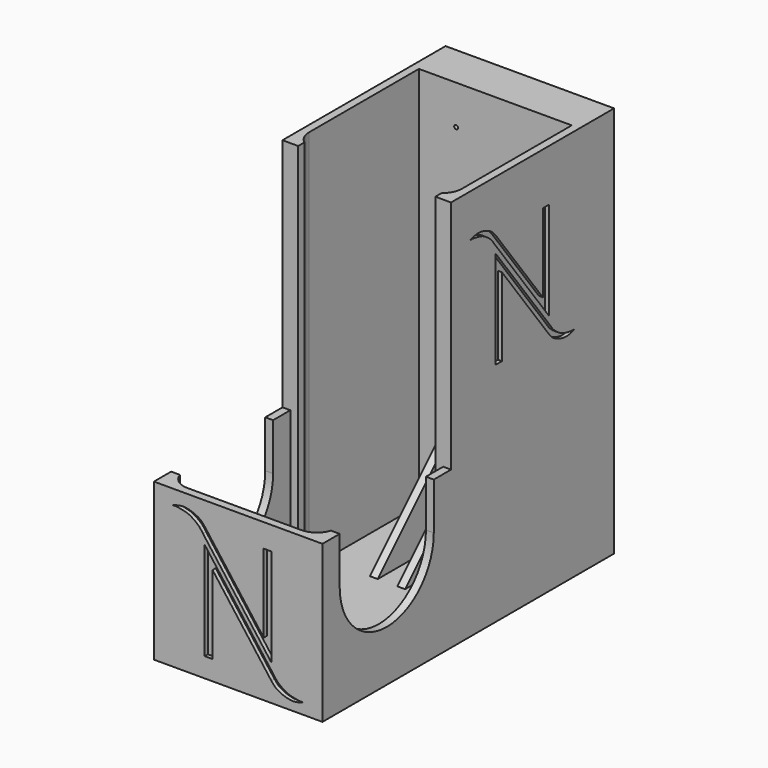
from build123d import *

# Parameters (mm, degrees)
F0_W         = 43
F0_H         = 84
F1_DEPTH     = 100
F2_W         = 43
F2_H         = 41
F3_DEPTH     = 60
F4_W         = 39
F4_H         = 39
F5_DEPTH     = 38
F6_W         = 39
F6_H         = 39
F7_DEPTH     = 98
F8_W         = 35
F8_H         = 2
F9_DEPTH     = 98
F10_T1_DEPTH = 98
F12_DEPTH    = 43
F13_R        = 5
F14_DEPTH    = 3
F15_R        = 5.5
F16_DEPTH    = 3
F17_W        = 2
F17_H        = 30
F18_DEPTH    = 30
F19_SIZE     = 29.99999
F21_DEPTH    = 1
F23_DEPTH    = 1
F25_DEPTH    = 1
F26_R        = 0.5
F27_DEPTH    = 2
F28_R        = 0.5
F29_DEPTH    = 2
F30_DEPTH    = 6
F31_DEPTH    = 6
F32_DEPTH    = 6
F33_R        = 0.5
F34_DEPTH    = 2
F35_R        = 0.5
F36_DEPTH    = 2
F37_DEPTH    = 6
F38_DEPTH    = 6


# Not quite as in the source:
# - a fillet or chamfer that OpenCascade refuses, or shapes differently, is made with other operations: its cross-section is extruded or revolved along the edge and cut away or added
# - a fillet or chamfer is up to 0.001 mm smaller than in the source, because OpenCascade refuses the exact size


with BuildPart() as f1:
    # F0 (on Top) → F1 (new body)
    with BuildSketch(Plane.XY):
        Rectangle(F0_W, F0_H)
    extrude(amount=F1_DEPTH)

    # F2 (on face) → F3 (cut)
    with BuildSketch(Plane.XY.offset(100)):
        with Locations((0, -21.5)):
            Rectangle(F2_W, F2_H)
    extrude(amount=-F3_DEPTH, mode=Mode.SUBTRACT)

    # F4 (on face) → F5 (cut)
    with BuildSketch(Plane.XY.offset(40)):
        with Locations((0, -20.5)):
            Rectangle(F4_W, F4_H)
    extrude(amount=-F5_DEPTH, mode=Mode.SUBTRACT)

    # F6 (on face) → F7 (cut)
    with BuildSketch(Plane.XY.offset(100)):
        with Locations((0, 20.5)):
            Rectangle(F6_W, F6_H)
    extrude(amount=-F7_DEPTH, mode=Mode.SUBTRACT)

    # F8 (on face) → F9 (cut)
    with BuildSketch(Plane.XY.offset(100)):
        Rectangle(F8_W, F8_H)
    extrude(amount=-F9_DEPTH, mode=Mode.SUBTRACT)

    # F10: fillet of radius 5 on 2 edges, made by hand

    # F10_s2 → F10_t1 (join)
    with BuildSketch(Plane.XY.offset(2)):
        with BuildLine():
            ThreePointArc((-19.5, 5), (-18.972135955, 2.7639320225), (-17.5, 1))
            Line((-17.5, 1), (-19.5, 1))
            Line((-19.5, 1), (-19.5, 5))
        make_face()
        with BuildLine():
            ThreePointArc((17.5, 1), (18.972135955, 2.7639320225), (19.5, 5))
            Line((19.5, 5), (19.5, 1))
            Line((19.5, 1), (17.5, 1))
        make_face()
    extrude(amount=F10_T1_DEPTH)

    # F11 (on face) → F12 (cut)
    with BuildSketch(Plane(origin=(-21.5, 0, 0), x_dir=(0, -1, 0), z_dir=(-1, 0, 0))):
        with BuildLine():
            Line((6.5, 40), (6.5, 28))
            ThreePointArc((6.5, 28), (21.5, 13), (36.5, 28))
            Line((36.5, 28), (36.5, 40))
            Line((36.5, 40), (6.5, 40))
        make_face()
    extrude(amount=-F12_DEPTH, mode=Mode.SUBTRACT)

    # F13
    f13_edges = [f1.edges().sort_by_distance(p)[0] for p in [
        (-19.5, -40, 21),
        (19.5, -40, 21),
    ]]
    fillet(f13_edges, radius=F13_R)

    # F14 (add): a face of the model
    f14_faces = [f1.faces().sort_by_distance(p)[0] for p in [
        (0, 42, 50),
    ]]
    extrude(f14_faces, amount=F14_DEPTH)

    # F15 (on face) → F16 (cut)
    with BuildSketch(Plane(origin=(0, 45, 0), x_dir=(-1, 0, 0), z_dir=(0, 1, 0))):
        with Locations((10, 90)):
            Circle(F15_R)
        with Locations((-10, 90)):
            Circle(F15_R)
        with Locations((-10, 10)):
            Circle(F15_R)
        with Locations((10, 10)):
            Circle(F15_R)
    extrude(amount=-F16_DEPTH, mode=Mode.SUBTRACT)

    # F17 (on face) → F18 (join)
    with BuildSketch(Plane.XY.offset(2)):
        with Locations((0, 25)):
            Rectangle(F17_W, F17_H)
        with Locations((7, 25)):
            Rectangle(F17_W, F17_H)
        with Locations((-7, 25)):
            Rectangle(F17_W, F17_H)
    extrude(amount=F18_DEPTH)

    # F19 (size 30 in the source; OpenCascade refuses exactly that, so slightly less here)
    f19_edges = [f1.edges().sort_by_distance(p)[0] for p in [
        (-7, 10, 32),
        (0, 10, 32),
        (7, 10, 32),
    ]]
    chamfer(f19_edges, length=F19_SIZE)

    # F20 (on face) → F21 (cut)
    with BuildSketch(Plane.YZ.offset(21.5)):
        with BuildLine():
            Line((30.7126875989, 59.4153521478), (13.203869056, 82.7604435384))
            Line((13.203869056, 82.7604435384), (13.203869056, 57.7604435384))
            Line((13.203869056, 57.7604435384), (15.203869056, 57.7604435384))
            Line((15.203869056, 57.7604435384), (15.203869056, 77.7604435384))
            Line((15.203869056, 77.7604435384), (30.203869056, 57.7604435384))
            add(Edge.make_bspline(
                [(30.203869056, 57.7604435384), (30.5911530821, 57.276545428), (31.4156642738, 56.2463469671), (33.7048595404, 55.2813534719), (35.8930037718, 54.7622938939), (37.6230920038, 55.2732884025), (38.5322710667, 55.5418212437)],
                knots=[0, 0, 0, 0, 0.2269766379, 0.4832235918, 0.7284287114, 1, 1, 1, 1], degree=3))
            add(Edge.make_bspline(
                [(38.5322710667, 55.5418212437), (38.1831508623, 55.5237925594), (37.4110779588, 55.4839224558), (35.8091615291, 55.8243371923), (34.4178365647, 56.1496791023), (33.0309594623, 56.9804929726), (31.5764378105, 58.1302638948), (30.9915396307, 59.0004758727), (30.7126875989, 59.4153521478)],
                knots=[0, 0, 0, 0, 0.1423640494, 0.3148354738, 0.477082541, 0.6483059214, 0.8323287509, 1, 1, 1, 1], degree=3))
        make_face()
        with BuildLine():
            Line((12.7480653018, 85.1540187478), (30.2568838447, 61.8089273572))
            Line((30.2568838447, 61.8089273572), (30.2568838447, 86.8089273572))
            Line((30.2568838447, 86.8089273572), (28.2568838447, 86.8089273572))
            Line((28.2568838447, 86.8089273572), (28.2568838447, 66.8089273572))
            Line((28.2568838447, 66.8089273572), (13.2568838447, 86.8089273572))
            add(Edge.make_bspline(
                [(13.2568838447, 86.8089273572), (12.8695998186, 87.2928254676), (12.0450886269, 88.3230239285), (9.7558933603, 89.2880174237), (7.5677491289, 89.8070770017), (5.8376608969, 89.2960824931), (4.928481834, 89.0275496519)],
                knots=[0, 0, 0, 0, 0.2269766379, 0.4832235918, 0.7284287114, 1, 1, 1, 1], degree=3))
            add(Edge.make_bspline(
                [(4.928481834, 89.0275496519), (5.2776020384, 89.0455783363), (6.0496749419, 89.0854484398), (7.6515913716, 88.7450337033), (9.042916336, 88.4196917933), (10.4297934384, 87.5888779231), (11.8843150902, 86.4391070008), (12.46921327, 85.5688950229), (12.7480653018, 85.1540187478)],
                knots=[0, 0, 0, 0, 0.1423640494, 0.3148354738, 0.477082541, 0.6483059214, 0.8323287509, 1, 1, 1, 1], degree=3))
        make_face()
    extrude(amount=-F21_DEPTH, mode=Mode.SUBTRACT)

    # F22 (on face) → F23 (cut)
    with BuildSketch(Plane(origin=(-21.5, 0, 0), x_dir=(0, -1, 0), z_dir=(-1, 0, 0))):
        with BuildLine():
            Line((-12.7911877275, 60.483143282), (-30.3000062704, 83.8282346725))
            Line((-30.3000062704, 83.8282346725), (-30.3000062704, 58.8282346725))
            Line((-30.3000062704, 58.8282346725), (-28.3000062704, 58.8282346725))
            Line((-28.3000062704, 58.8282346725), (-28.3000062704, 78.8282346725))
            Line((-28.3000062704, 78.8282346725), (-13.3000062704, 58.8282346725))
            add(Edge.make_bspline(
                [(-13.3000062704, 58.8282346725), (-12.9127222442, 58.3443365621), (-12.0882110526, 57.3141381012), (-9.799015786, 56.349144606), (-7.6108715546, 55.830085028), (-5.8807833225, 56.3410795367), (-4.9716042597, 56.6096123778)],
                knots=[0, 0, 0, 0, 0.2269766379, 0.4832235918, 0.7284287114, 1, 1, 1, 1], degree=3))
            add(Edge.make_bspline(
                [(-4.9716042597, 56.6096123778), (-5.320724464, 56.5915836935), (-6.0927973675, 56.5517135899), (-7.6947137972, 56.8921283264), (-9.0860387617, 57.2174702364), (-10.4729158641, 58.0482841067), (-11.9274375159, 59.1980550289), (-12.5123356957, 60.0682670068), (-12.7911877275, 60.483143282)],
                knots=[0, 0, 0, 0, 0.1423640494, 0.3148354738, 0.477082541, 0.6483059214, 0.8323287509, 1, 1, 1, 1], degree=3))
        make_face()
        with BuildLine():
            Line((-30.7558100246, 86.2218098819), (-13.2469914816, 62.8767184913))
            Line((-13.2469914816, 62.8767184913), (-13.2469914816, 87.8767184913))
            Line((-13.2469914816, 87.8767184913), (-15.2469914816, 87.8767184913))
            Line((-15.2469914816, 87.8767184913), (-15.2469914816, 67.8767184913))
            Line((-15.2469914816, 67.8767184913), (-30.2469914816, 87.8767184913))
            add(Edge.make_bspline(
                [(-30.2469914816, 87.8767184913), (-30.6342755078, 88.3606166017), (-31.4587866995, 89.3908150626), (-33.747981966, 90.3558085578), (-35.9361261975, 90.8748681358), (-37.6662144295, 90.3638736272), (-38.5753934924, 90.095340786)],
                knots=[0, 0, 0, 0, 0.2269766379, 0.4832235918, 0.7284287114, 1, 1, 1, 1], degree=3))
            add(Edge.make_bspline(
                [(-38.5753934924, 90.095340786), (-38.226273288, 90.1133694704), (-37.4542003845, 90.1532395739), (-35.8522839548, 89.8128248375), (-34.4609589904, 89.4874829274), (-33.074081888, 88.6566690572), (-31.6195602362, 87.5068981349), (-31.0346620564, 86.636686157), (-30.7558100246, 86.2218098819)],
                knots=[0, 0, 0, 0, 0.1423640494, 0.3148354738, 0.477082541, 0.6483059214, 0.8323287509, 1, 1, 1, 1], degree=3))
        make_face()
    extrude(amount=-F23_DEPTH, mode=Mode.SUBTRACT)

    # F24 (on face) → F25 (cut)
    with BuildSketch(Plane.XZ.offset(42)):
        with BuildLine():
            Line((8.9712467361, 6.654908032), (-8.5375718068, 29.9999994226))
            Line((-8.5375718068, 29.9999994226), (-8.5375718068, 4.9999994226))
            Line((-8.5375718068, 4.9999994226), (-6.5375718068, 4.9999994226))
            Line((-6.5375718068, 4.9999994226), (-6.5375718068, 24.9999994226))
            Line((-6.5375718068, 24.9999994226), (8.4624281932, 4.9999994226))
            add(Edge.make_bspline(
                [(8.4624281932, 4.9999994226), (8.8497122193, 4.5161013121), (9.674223411, 3.4859028513), (11.9634186776, 2.5209093561), (14.151562909, 2.0018497781), (15.8816511411, 2.5128442867), (16.7908302039, 2.7813771279)],
                knots=[0, 0, 0, 0, 0.2269766379, 0.4832235918, 0.7284287114, 1, 1, 1, 1], degree=3))
            add(Edge.make_bspline(
                [(16.7908302039, 2.7813771279), (16.4417099996, 2.7633484435), (15.669637096, 2.72347834), (14.0677206663, 3.0638930764), (12.6763957019, 3.3892349865), (11.2895185995, 4.2200488567), (9.8349969477, 5.369819779), (9.2500987679, 6.2400317569), (8.9712467361, 6.654908032)],
                knots=[0, 0, 0, 0, 0.1423640494, 0.3148354738, 0.477082541, 0.6483059214, 0.8323287509, 1, 1, 1, 1], degree=3))
        make_face()
        with BuildLine():
            Line((-8.993375561, 32.3935746319), (8.515442982, 9.0484832413))
            Line((8.515442982, 9.0484832413), (8.515442982, 34.0484832413))
            Line((8.515442982, 34.0484832413), (6.515442982, 34.0484832413))
            Line((6.515442982, 34.0484832413), (6.515442982, 14.0484832413))
            Line((6.515442982, 14.0484832413), (-8.484557018, 34.0484832413))
            add(Edge.make_bspline(
                [(-8.484557018, 34.0484832413), (-8.8718410442, 34.5323813518), (-9.6963522359, 35.5625798127), (-11.9855475024, 36.5275733078), (-14.1736917339, 37.0466328859), (-15.9037799659, 36.5356383772), (-16.8129590288, 36.267105536)],
                knots=[0, 0, 0, 0, 0.2269766379, 0.4832235918, 0.7284287114, 1, 1, 1, 1], degree=3))
            add(Edge.make_bspline(
                [(-16.8129590288, 36.267105536), (-16.4638388244, 36.2851342204), (-15.6917659209, 36.325004324), (-14.0898494912, 35.9845895875), (-12.6985245268, 35.6592476775), (-11.3116474244, 34.8284338072), (-9.8571257726, 33.678662885), (-9.2722275928, 32.808450907), (-8.993375561, 32.3935746319)],
                knots=[0, 0, 0, 0, 0.1423640494, 0.3148354738, 0.477082541, 0.6483059214, 0.8323287509, 1, 1, 1, 1], degree=3))
        make_face()
    extrude(amount=-F25_DEPTH, mode=Mode.SUBTRACT)

    # F26 (on face) → F27 (cut)
    with BuildSketch(Plane(origin=(0, 42, 0), x_dir=(-1, 0, 0), z_dir=(0, 1, 0))):
        with Locations((-10, 90)):
            Circle(F26_R)
    extrude(amount=-F27_DEPTH, mode=Mode.SUBTRACT)

    # F28 (on face) → F29 (cut)
    with BuildSketch(Plane(origin=(0, 42, 0), x_dir=(-1, 0, 0), z_dir=(0, 1, 0))):
        with Locations((10, 90)):
            Circle(F28_R)
    extrude(amount=-F29_DEPTH, mode=Mode.SUBTRACT)

    # F30 (add): a face of the model
    f30_faces = [f1.faces().sort_by_distance(p)[0] for p in [
        (0, 45, 50),
    ]]
    extrude(f30_faces, amount=F30_DEPTH)

    # F31 (add): a face of the model
    f31_faces = [f1.faces().sort_by_distance(p)[0] for p in [
        (15.3444365081, 42, 90),
    ]]
    extrude(f31_faces, amount=F31_DEPTH)

    # F32 (add): a face of the model
    f32_faces = [f1.faces().sort_by_distance(p)[0] for p in [
        (-4.6555634919, 42, 90),
    ]]
    extrude(f32_faces, amount=F32_DEPTH)

    # F33 (on face) → F34 (cut)
    with BuildSketch(Plane(origin=(0, 42, 0), x_dir=(-1, 0, 0), z_dir=(0, 1, 0))):
        with Locations((-10, 10)):
            Circle(F33_R)
    extrude(amount=-F34_DEPTH, mode=Mode.SUBTRACT)

    # F35 (on face) → F36 (cut)
    with BuildSketch(Plane(origin=(0, 42, 0), x_dir=(-1, 0, 0), z_dir=(0, 1, 0))):
        with Locations((10, 10)):
            Circle(F35_R)
    extrude(amount=-F36_DEPTH, mode=Mode.SUBTRACT)

    # F37 (add): a face of the model
    f37_faces = [f1.faces().sort_by_distance(p)[0] for p in [
        (15.3444365081, 42, 10),
    ]]
    extrude(f37_faces, amount=F37_DEPTH)

    # F38 (add): a face of the model
    f38_faces = [f1.faces().sort_by_distance(p)[0] for p in [
        (-4.6555634919, 42, 10),
    ]]
    extrude(f38_faces, amount=F38_DEPTH)


solid = f1.part
